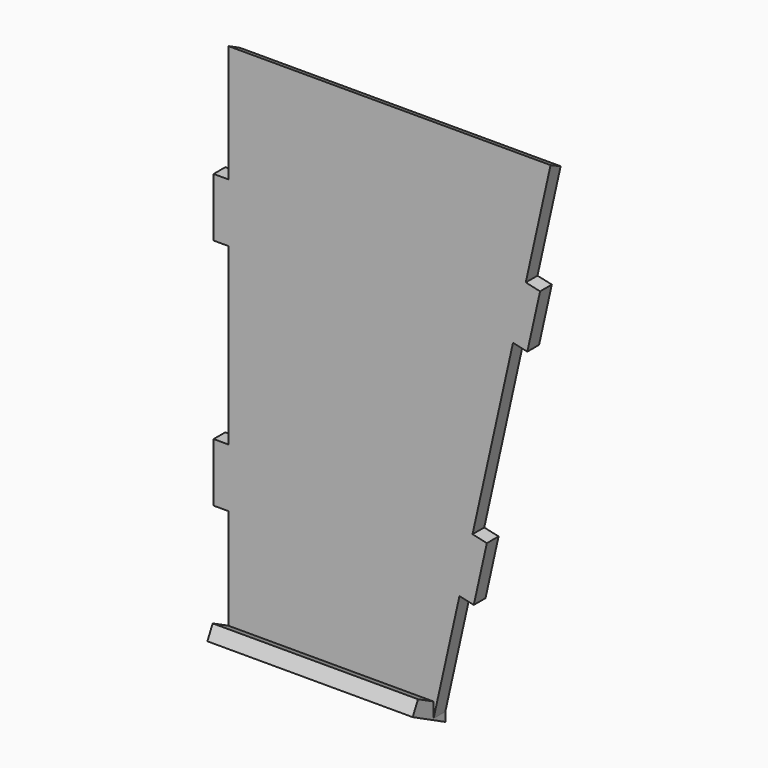
from build123d import *

# Parameters (mm, degrees)
F1_DEPTH = 3.175
F3_DEPTH = 43.942
F5_DEPTH = 76.2
F6_DEPTH = 44.45


# Not quite as in the source:
# - a feature names something its author has since deleted; it is built from what else it names


with BuildPart() as f1:
    # F0 (on Front) → F1 (new body)
    with BuildSketch(Plane.XZ):
        Polygon((-34.925, -57.0107064), (9.4471751978, -57.0107064), (15.1238233026, -31.5280514049), (18.2228604819, -32.2184089652), (21.0519782071, -19.5184089652), (17.9529410277, -18.8280514049), (26.7166720978, 20.512617808), (29.8157092771, 19.8222602477), (32.5771395181, 32.2184089652), (29.4781023387, 32.9087665254), (34.8471751978, 57.0107064), (-34.925, 57.0107064), (-34.925, 31.6107064), (-38.1, 31.6107064), (-38.1, 18.9107064), (-34.925, 18.9107064), (-34.925, -18.9107064), (-38.1, -18.9107064), (-38.1, -31.6107064), (-34.925, -31.6107064), align=None)
    extrude(amount=F1_DEPTH)

    # F2 (on face) → F3 (join)
    with BuildSketch(Plane(origin=(-34.925, 0, 0), x_dir=(0, -1, 0), z_dir=(-1, 0, 0))):
        Polygon((0, -58.6279720227), (3.175, -57.0107064), (8.8332357394, -54.1285425744), (7.3921538265, -51.2994247047), (0, -55.0648030547), align=None)
    extrude(amount=-F3_DEPTH)

    # F4 (on face) → F5 (cut)
    with BuildSketch(Plane(origin=(-34.925, 0, 0), x_dir=(0, -1, 0), z_dir=(-1, 0, 0))):
        Polygon((0, 55.3934407773), (3.175, 57.0107064), (0, 57.0107064), align=None)
    extrude(amount=-F5_DEPTH, mode=Mode.SUBTRACT)

    # F2 (on face) → F6 (join)
    with BuildSketch(Plane(origin=(-34.925, 0, 0), x_dir=(0, -1, 0), z_dir=(-1, 0, 0))):
        Polygon((0, -58.6279720227), (3.175, -57.0107064), (8.8332357394, -54.1285425744), (7.3921538265, -51.2994247047), (0, -55.0648030547), align=None)
    extrude(amount=-F6_DEPTH)


solid = f1.part
